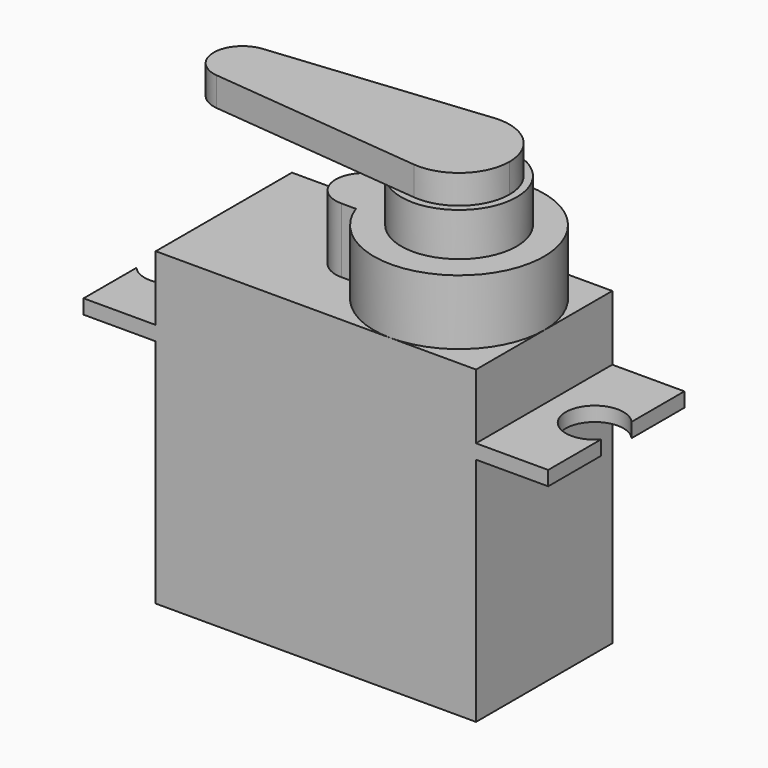
from build123d import *

# Parameters (mm, degrees)
F0_W      = 22.2
F0_H      = 11.8
F1_DEPTH  = 21.5
F5_DEPTH  = 4.5
F6_DEPTH  = 1
F7_R      = 4
F8_DEPTH  = 3
F10_DEPTH = 2


# Not quite as in the source:
# - a pattern or mirror of a feature is missing from the dataset's text; its kind, count and spacing are read off the source's solid


with BuildPart() as f1:
    # F0 (on Top) → F1 (new body)
    with BuildSketch(Plane.XY):
        Rectangle(F0_W, F0_H)
    extrude(amount=F1_DEPTH)

    # F4 (on face) → F5 (join)
    with BuildSketch(Plane.XY.offset(21.5)):
        with BuildLine():
            Line((-1.3506756346, -2), (-0.3506756346, -2))
            ThreePointArc((-0.3506756346, -2), (11.1, 0), (-0.3506756346, 2))
            Line((-0.3506756346, 2), (-1.3506756346, 2))
            ThreePointArc((-1.3506756346, 2), (-3.3506756346, 0), (-1.3506756346, -2))
        make_face()
    extrude(amount=F5_DEPTH)

    # F3 (on offset) → F6 (join)
    with BuildSketch(Plane.XY.offset(16)):
        with BuildLine():
            Line((16.1, 5.9), (11.1, 5.9))
            Line((11.1, 5.9), (11.1, -5.9))
            Line((11.1, -5.9), (16.1, -5.9))
            Line((16.1, -5.9), (16.1, -1.3228756555))
            ThreePointArc((16.1, -1.3228756555), (12.6, 0), (16.1, 1.3228756555))
            Line((16.1, 1.3228756555), (16.1, 5.9))
        make_face()
    f6 = extrude(amount=F6_DEPTH)

    # F6_copies: F6 across plane
    add(f6.mirror(Plane(origin=(0, 0, 0), x_dir=(0, 0, -1), z_dir=(-1, 0, 0))))


with BuildPart() as f8:
    # F7 (on face) → F8 (new body)
    with BuildSketch(Plane.XY.offset(26)):
        with Locations((5.2, 0)):
            Circle(F7_R)
    extrude(amount=F8_DEPTH)

    # F9 (on face) → F10 (join)
    with BuildSketch(Plane.XY.offset(29)):
        with BuildLine():
            ThreePointArc((4.85, -3.4824560299), (7.5478713764, -2.5956694705), (8.7, 0))
            ThreePointArc((8.7, 0), (7.5478713764, 2.5956694705), (4.85, 3.4824560299))
            ThreePointArc((4.85, 3.4824560299), (1.7, 0), (4.85, -3.4824560299))
        make_face()
        with BuildLine():
            ThreePointArc((4.85, -3.4824560299), (1.7, 0), (4.85, 3.4824560299))
            Line((4.85, 3.4824560299), (-10, 1.9899748742))
            ThreePointArc((-10, 1.9899748742), (-11.8, 0), (-10, -1.9899748742))
            Line((-10, -1.9899748742), (4.85, -3.4824560299))
        make_face()
    extrude(amount=F10_DEPTH)


solid = Compound([f1.part, f8.part])
